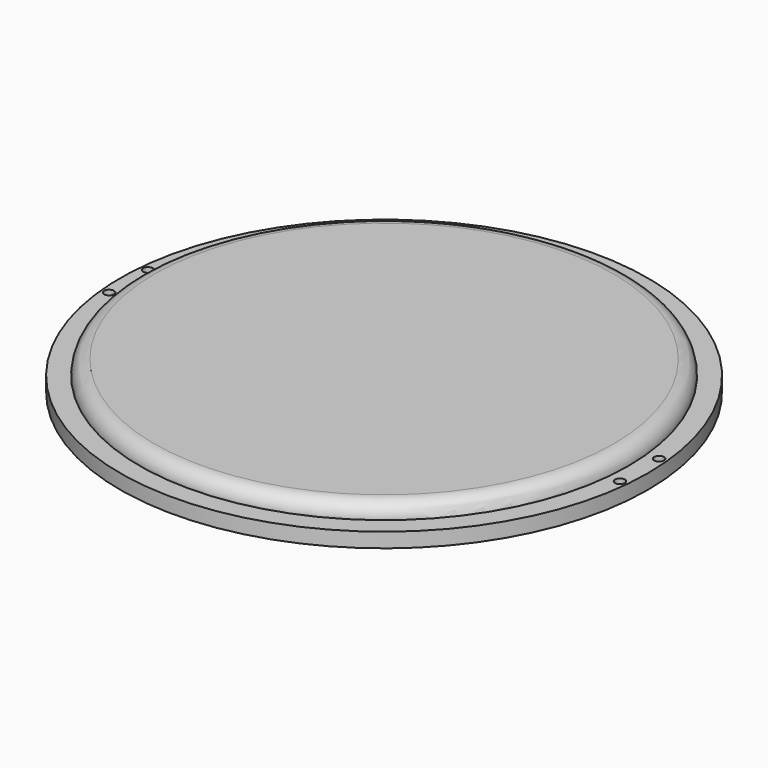
from build123d import *

# Parameters (mm, degrees)
F0_R     = 54
F1_DEPTH = 3
F2_R     = 50
F3_DEPTH = 3
F4_R     = 2.99999
F5_R     = 1
F6_DEPTH = 3


# Not quite as in the source:
# - a fillet or chamfer is up to 0.001 mm smaller than in the source, because OpenCascade refuses the exact size


with BuildPart() as f1:
    # F0 (on Top) → F1 (new body)
    with BuildSketch(Plane.XY):
        Circle(F0_R)
    extrude(amount=F1_DEPTH)

    # F5 (on face) → F6 (cut, through all)
    with BuildSketch(Plane(origin=(0, 0, 0), x_dir=(1, 0, 0), z_dir=(0, 0, -1))):
        with Locations((-52.2613624009, 5)):
            Circle(F5_R)
        with Locations((-52.2613624009, -5)):
            Circle(F5_R)
        with Locations((52.2613624009, -5)):
            Circle(F5_R)
        with Locations((52.2613624009, 5)):
            Circle(F5_R)
    extrude(amount=-F6_DEPTH, mode=Mode.SUBTRACT)


with BuildPart() as f3:
    # F2 (on face) → F3 (new body)
    with BuildSketch(Plane.XY.offset(3)):
        Circle(F2_R)
    extrude(amount=F3_DEPTH)

    # F4 (radius 3 in the source; OpenCascade refuses exactly that, so slightly less here)
    f4_edges = [f3.edges().sort_by_distance(p)[0] for p in [
        (-50, 0, 6),
    ]]
    fillet(f4_edges, radius=F4_R)


solid = Compound([f1.part, f3.part])
